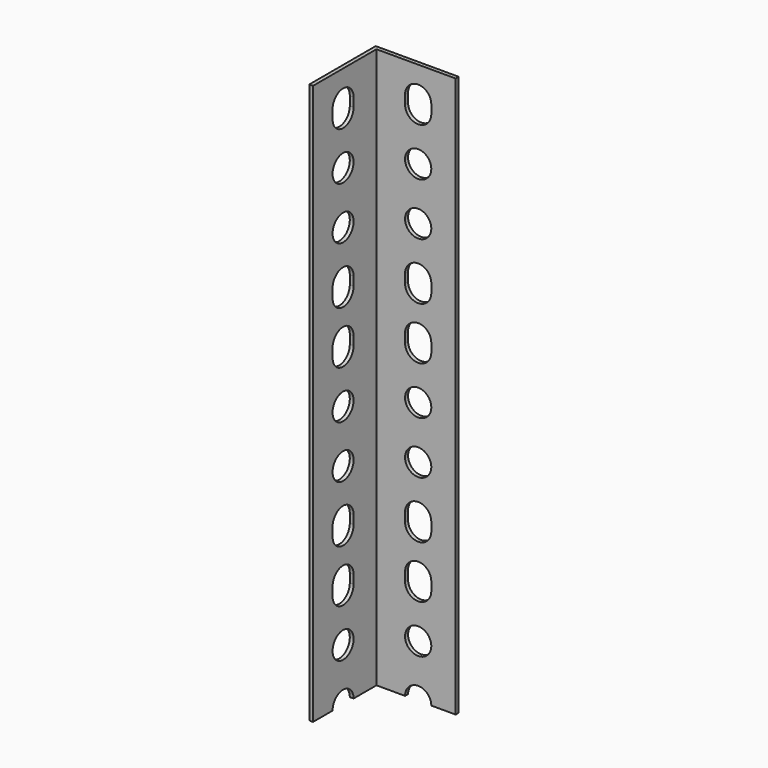
from build123d import *

# Parameters (mm, degrees)
F2_DEPTH = 203.2
F3_R     = 4.7625
F5_DEPTH = 1.3726
F4_R     = 4.7625
F6_DEPTH = 1.3726


# Not quite as in the source:
# - a variable given as a bare number and used for a length is read in inches; the dataset says mm whatever the document's units were


with BuildPart() as f2:
    # F1 (on Top) → F2 (new body)
    with BuildSketch(Plane.XY):
        Polygon((-1.3716, 1.3716), (-1.3716, -28.7528), (0, -28.7528), (0, 0), (28.7528, 0), (28.7528, 1.3716), align=None)
    extrude(amount=F2_DEPTH)

    # F3 (on face) → F5 (cut, through all)
    with BuildSketch(Plane.XZ):
        with Locations((15.1384, 19.05)):
            Circle(F3_R)
        with Locations((15.1384, 0)):
            Circle(F3_R)
        with BuildLine():
            Line((19.9009, 36.5125), (19.9009, 39.6875))
            ThreePointArc((19.9009, 39.6875), (15.1384, 44.45), (10.3759, 39.6875))
            Line((10.3759, 39.6875), (10.3759, 36.5125))
            ThreePointArc((10.3759, 36.5125), (15.1384, 31.75), (19.9009, 36.5125))
        make_face()
        with BuildLine():
            Line((19.9009, 55.5625), (19.9009, 58.7375))
            ThreePointArc((19.9009, 58.7375), (15.1384, 63.5), (10.3759, 58.7375))
            Line((10.3759, 58.7375), (10.3759, 55.5625))
            ThreePointArc((10.3759, 55.5625), (15.1384, 50.8), (19.9009, 55.5625))
        make_face()
        with BuildLine():
            Line((19.9009, 131.7625), (19.9009, 134.9375))
            ThreePointArc((19.9009, 134.9375), (15.1384, 139.7), (10.3759, 134.9375))
            Line((10.3759, 134.9375), (10.3759, 131.7625))
            ThreePointArc((10.3759, 131.7625), (15.1384, 127), (19.9009, 131.7625))
        make_face()
        with Locations((15.1384, 95.25)):
            Circle(F3_R)
        with Locations((15.1384, 76.2)):
            Circle(F3_R)
        with BuildLine():
            Line((19.9009, 112.7125), (19.9009, 115.8875))
            ThreePointArc((19.9009, 115.8875), (15.1384, 120.65), (10.3759, 115.8875))
            Line((10.3759, 115.8875), (10.3759, 112.7125))
            ThreePointArc((10.3759, 112.7125), (15.1384, 107.95), (19.9009, 112.7125))
        make_face()
        with BuildLine():
            Line((19.9009, 207.9625), (19.9009, 211.1375))
            ThreePointArc((19.9009, 211.1375), (15.1384, 215.9), (10.3759, 211.1375))
            Line((10.3759, 211.1375), (10.3759, 207.9625))
            ThreePointArc((10.3759, 207.9625), (15.1384, 203.2), (19.9009, 207.9625))
        make_face()
        with Locations((15.1384, 171.45)):
            Circle(F3_R)
        with Locations((15.1384, 152.4)):
            Circle(F3_R)
        with BuildLine():
            Line((19.9009, 188.9125), (19.9009, 192.0875))
            ThreePointArc((19.9009, 192.0875), (15.1384, 196.85), (10.3759, 192.0875))
            Line((10.3759, 192.0875), (10.3759, 188.9125))
            ThreePointArc((10.3759, 188.9125), (15.1384, 184.15), (19.9009, 188.9125))
        make_face()
        with BuildLine():
            Line((19.9009, 284.1625), (19.9009, 287.3375))
            ThreePointArc((19.9009, 287.3375), (15.1384, 292.1), (10.3759, 287.3375))
            Line((10.3759, 287.3375), (10.3759, 284.1625))
            ThreePointArc((10.3759, 284.1625), (15.1384, 279.4), (19.9009, 284.1625))
        make_face()
        with Locations((15.1384, 247.65)):
            Circle(F3_R)
        with Locations((15.1384, 228.6)):
            Circle(F3_R)
        with BuildLine():
            Line((19.9009, 265.1125), (19.9009, 268.2875))
            ThreePointArc((19.9009, 268.2875), (15.1384, 273.05), (10.3759, 268.2875))
            Line((10.3759, 268.2875), (10.3759, 265.1125))
            ThreePointArc((10.3759, 265.1125), (15.1384, 260.35), (19.9009, 265.1125))
        make_face()
        with BuildLine():
            Line((19.9009, 360.3625), (19.9009, 363.5375))
            ThreePointArc((19.9009, 363.5375), (15.1384, 368.3), (10.3759, 363.5375))
            Line((10.3759, 363.5375), (10.3759, 360.3625))
            ThreePointArc((10.3759, 360.3625), (15.1384, 355.6), (19.9009, 360.3625))
        make_face()
        with Locations((15.1384, 323.85)):
            Circle(F3_R)
        with Locations((15.1384, 304.8)):
            Circle(F3_R)
        with BuildLine():
            Line((19.9009, 341.3125), (19.9009, 344.4875))
            ThreePointArc((19.9009, 344.4875), (15.1384, 349.25), (10.3759, 344.4875))
            Line((10.3759, 344.4875), (10.3759, 341.3125))
            ThreePointArc((10.3759, 341.3125), (15.1384, 336.55), (19.9009, 341.3125))
        make_face()
        with BuildLine():
            Line((19.9009, 436.5625), (19.9009, 439.7375))
            ThreePointArc((19.9009, 439.7375), (15.1384, 444.5), (10.3759, 439.7375))
            Line((10.3759, 439.7375), (10.3759, 436.5625))
            ThreePointArc((10.3759, 436.5625), (15.1384, 431.8), (19.9009, 436.5625))
        make_face()
        with Locations((15.1384, 400.05)):
            Circle(F3_R)
        with Locations((15.1384, 381)):
            Circle(F3_R)
        with BuildLine():
            Line((19.9009, 417.5125), (19.9009, 420.6875))
            ThreePointArc((19.9009, 420.6875), (15.1384, 425.45), (10.3759, 420.6875))
            Line((10.3759, 420.6875), (10.3759, 417.5125))
            ThreePointArc((10.3759, 417.5125), (15.1384, 412.75), (19.9009, 417.5125))
        make_face()
        with BuildLine():
            Line((19.9009, 512.7625), (19.9009, 515.9375))
            ThreePointArc((19.9009, 515.9375), (15.1384, 520.7), (10.3759, 515.9375))
            Line((10.3759, 515.9375), (10.3759, 512.7625))
            ThreePointArc((10.3759, 512.7625), (15.1384, 508), (19.9009, 512.7625))
        make_face()
        with Locations((15.1384, 476.25)):
            Circle(F3_R)
        with Locations((15.1384, 457.2)):
            Circle(F3_R)
        with BuildLine():
            Line((19.9009, 493.7125), (19.9009, 496.8875))
            ThreePointArc((19.9009, 496.8875), (15.1384, 501.65), (10.3759, 496.8875))
            Line((10.3759, 496.8875), (10.3759, 493.7125))
            ThreePointArc((10.3759, 493.7125), (15.1384, 488.95), (19.9009, 493.7125))
        make_face()
        with BuildLine():
            Line((19.9009, 588.9625), (19.9009, 592.1375))
            ThreePointArc((19.9009, 592.1375), (15.1384, 596.9), (10.3759, 592.1375))
            Line((10.3759, 592.1375), (10.3759, 588.9625))
            ThreePointArc((10.3759, 588.9625), (15.1384, 584.2), (19.9009, 588.9625))
        make_face()
        with Locations((15.1384, 552.45)):
            Circle(F3_R)
        with Locations((15.1384, 533.4)):
            Circle(F3_R)
        with BuildLine():
            Line((19.9009, 569.9125), (19.9009, 573.0875))
            ThreePointArc((19.9009, 573.0875), (15.1384, 577.85), (10.3759, 573.0875))
            Line((10.3759, 573.0875), (10.3759, 569.9125))
            ThreePointArc((10.3759, 569.9125), (15.1384, 565.15), (19.9009, 569.9125))
        make_face()
        with BuildLine():
            Line((19.9009, 665.1625), (19.9009, 668.3375))
            ThreePointArc((19.9009, 668.3375), (15.1384, 673.1), (10.3759, 668.3375))
            Line((10.3759, 668.3375), (10.3759, 665.1625))
            ThreePointArc((10.3759, 665.1625), (15.1384, 660.4), (19.9009, 665.1625))
        make_face()
        with Locations((15.1384, 628.65)):
            Circle(F3_R)
        with Locations((15.1384, 609.6)):
            Circle(F3_R)
        with BuildLine():
            Line((19.9009, 646.1125), (19.9009, 649.2875))
            ThreePointArc((19.9009, 649.2875), (15.1384, 654.05), (10.3759, 649.2875))
            Line((10.3759, 649.2875), (10.3759, 646.1125))
            ThreePointArc((10.3759, 646.1125), (15.1384, 641.35), (19.9009, 646.1125))
        make_face()
        with BuildLine():
            Line((19.9009, 741.3625), (19.9009, 744.5375))
            ThreePointArc((19.9009, 744.5375), (15.1384, 749.3), (10.3759, 744.5375))
            Line((10.3759, 744.5375), (10.3759, 741.3625))
            ThreePointArc((10.3759, 741.3625), (15.1384, 736.6), (19.9009, 741.3625))
        make_face()
        with Locations((15.1384, 704.85)):
            Circle(F3_R)
        with Locations((15.1384, 685.8)):
            Circle(F3_R)
        with BuildLine():
            Line((19.9009, 722.3125), (19.9009, 725.4875))
            ThreePointArc((19.9009, 725.4875), (15.1384, 730.25), (10.3759, 725.4875))
            Line((10.3759, 725.4875), (10.3759, 722.3125))
            ThreePointArc((10.3759, 722.3125), (15.1384, 717.55), (19.9009, 722.3125))
        make_face()
        with BuildLine():
            Line((19.9009, 817.5625), (19.9009, 820.7375))
            ThreePointArc((19.9009, 820.7375), (15.1384, 825.5), (10.3759, 820.7375))
            Line((10.3759, 820.7375), (10.3759, 817.5625))
            ThreePointArc((10.3759, 817.5625), (15.1384, 812.8), (19.9009, 817.5625))
        make_face()
        with Locations((15.1384, 781.05)):
            Circle(F3_R)
        with Locations((15.1384, 762)):
            Circle(F3_R)
        with BuildLine():
            Line((19.9009, 798.5125), (19.9009, 801.6875))
            ThreePointArc((19.9009, 801.6875), (15.1384, 806.45), (10.3759, 801.6875))
            Line((10.3759, 801.6875), (10.3759, 798.5125))
            ThreePointArc((10.3759, 798.5125), (15.1384, 793.75), (19.9009, 798.5125))
        make_face()
        with BuildLine():
            Line((19.9009, 893.7625), (19.9009, 896.9375))
            ThreePointArc((19.9009, 896.9375), (15.1384, 901.7), (10.3759, 896.9375))
            Line((10.3759, 896.9375), (10.3759, 893.7625))
            ThreePointArc((10.3759, 893.7625), (15.1384, 889), (19.9009, 893.7625))
        make_face()
        with Locations((15.1384, 857.25)):
            Circle(F3_R)
        with Locations((15.1384, 838.2)):
            Circle(F3_R)
        with BuildLine():
            Line((19.9009, 874.7125), (19.9009, 877.8875))
            ThreePointArc((19.9009, 877.8875), (15.1384, 882.65), (10.3759, 877.8875))
            Line((10.3759, 877.8875), (10.3759, 874.7125))
            ThreePointArc((10.3759, 874.7125), (15.1384, 869.95), (19.9009, 874.7125))
        make_face()
        with BuildLine():
            Line((19.9009, 969.9625), (19.9009, 973.1375))
            ThreePointArc((19.9009, 973.1375), (15.1384, 977.9), (10.3759, 973.1375))
            Line((10.3759, 973.1375), (10.3759, 969.9625))
            ThreePointArc((10.3759, 969.9625), (15.1384, 965.2), (19.9009, 969.9625))
        make_face()
        with Locations((15.1384, 933.45)):
            Circle(F3_R)
        with Locations((15.1384, 914.4)):
            Circle(F3_R)
        with BuildLine():
            Line((19.9009, 950.9125), (19.9009, 954.0875))
            ThreePointArc((19.9009, 954.0875), (15.1384, 958.85), (10.3759, 954.0875))
            Line((10.3759, 954.0875), (10.3759, 950.9125))
            ThreePointArc((10.3759, 950.9125), (15.1384, 946.15), (19.9009, 950.9125))
        make_face()
        with BuildLine():
            Line((19.9009, 1046.1625), (19.9009, 1049.3375))
            ThreePointArc((19.9009, 1049.3375), (15.1384, 1054.1), (10.3759, 1049.3375))
            Line((10.3759, 1049.3375), (10.3759, 1046.1625))
            ThreePointArc((10.3759, 1046.1625), (15.1384, 1041.4), (19.9009, 1046.1625))
        make_face()
        with Locations((15.1384, 1009.65)):
            Circle(F3_R)
        with Locations((15.1384, 990.6)):
            Circle(F3_R)
        with BuildLine():
            Line((19.9009, 1027.1125), (19.9009, 1030.2875))
            ThreePointArc((19.9009, 1030.2875), (15.1384, 1035.05), (10.3759, 1030.2875))
            Line((10.3759, 1030.2875), (10.3759, 1027.1125))
            ThreePointArc((10.3759, 1027.1125), (15.1384, 1022.35), (19.9009, 1027.1125))
        make_face()
        with BuildLine():
            Line((19.9009, 1122.3625), (19.9009, 1125.5375))
            ThreePointArc((19.9009, 1125.5375), (15.1384, 1130.3), (10.3759, 1125.5375))
            Line((10.3759, 1125.5375), (10.3759, 1122.3625))
            ThreePointArc((10.3759, 1122.3625), (15.1384, 1117.6), (19.9009, 1122.3625))
        make_face()
        with Locations((15.1384, 1085.85)):
            Circle(F3_R)
        with Locations((15.1384, 1066.8)):
            Circle(F3_R)
        with BuildLine():
            Line((19.9009, 1103.3125), (19.9009, 1106.4875))
            ThreePointArc((19.9009, 1106.4875), (15.1384, 1111.25), (10.3759, 1106.4875))
            Line((10.3759, 1106.4875), (10.3759, 1103.3125))
            ThreePointArc((10.3759, 1103.3125), (15.1384, 1098.55), (19.9009, 1103.3125))
        make_face()
        with BuildLine():
            Line((19.9009, 1198.5625), (19.9009, 1201.7375))
            ThreePointArc((19.9009, 1201.7375), (15.1384, 1206.5), (10.3759, 1201.7375))
            Line((10.3759, 1201.7375), (10.3759, 1198.5625))
            ThreePointArc((10.3759, 1198.5625), (15.1384, 1193.8), (19.9009, 1198.5625))
        make_face()
        with Locations((15.1384, 1162.05)):
            Circle(F3_R)
        with Locations((15.1384, 1143)):
            Circle(F3_R)
        with BuildLine():
            Line((19.9009, 1179.5125), (19.9009, 1182.6875))
            ThreePointArc((19.9009, 1182.6875), (15.1384, 1187.45), (10.3759, 1182.6875))
            Line((10.3759, 1182.6875), (10.3759, 1179.5125))
            ThreePointArc((10.3759, 1179.5125), (15.1384, 1174.75), (19.9009, 1179.5125))
        make_face()
        with BuildLine():
            Line((19.9009, 1274.7625), (19.9009, 1277.9375))
            ThreePointArc((19.9009, 1277.9375), (15.1384, 1282.7), (10.3759, 1277.9375))
            Line((10.3759, 1277.9375), (10.3759, 1274.7625))
            ThreePointArc((10.3759, 1274.7625), (15.1384, 1270), (19.9009, 1274.7625))
        make_face()
        with Locations((15.1384, 1238.25)):
            Circle(F3_R)
        with Locations((15.1384, 1219.2)):
            Circle(F3_R)
        with BuildLine():
            Line((19.9009, 1255.7125), (19.9009, 1258.8875))
            ThreePointArc((19.9009, 1258.8875), (15.1384, 1263.65), (10.3759, 1258.8875))
            Line((10.3759, 1258.8875), (10.3759, 1255.7125))
            ThreePointArc((10.3759, 1255.7125), (15.1384, 1250.95), (19.9009, 1255.7125))
        make_face()
        with BuildLine():
            Line((19.9009, 1350.9625), (19.9009, 1354.1375))
            ThreePointArc((19.9009, 1354.1375), (15.1384, 1358.9), (10.3759, 1354.1375))
            Line((10.3759, 1354.1375), (10.3759, 1350.9625))
            ThreePointArc((10.3759, 1350.9625), (15.1384, 1346.2), (19.9009, 1350.9625))
        make_face()
        with Locations((15.1384, 1314.45)):
            Circle(F3_R)
        with Locations((15.1384, 1295.4)):
            Circle(F3_R)
        with BuildLine():
            Line((19.9009, 1331.9125), (19.9009, 1335.0875))
            ThreePointArc((19.9009, 1335.0875), (15.1384, 1339.85), (10.3759, 1335.0875))
            Line((10.3759, 1335.0875), (10.3759, 1331.9125))
            ThreePointArc((10.3759, 1331.9125), (15.1384, 1327.15), (19.9009, 1331.9125))
        make_face()
        with BuildLine():
            Line((19.9009, 1427.1625), (19.9009, 1430.3375))
            ThreePointArc((19.9009, 1430.3375), (15.1384, 1435.1), (10.3759, 1430.3375))
            Line((10.3759, 1430.3375), (10.3759, 1427.1625))
            ThreePointArc((10.3759, 1427.1625), (15.1384, 1422.4), (19.9009, 1427.1625))
        make_face()
        with Locations((15.1384, 1390.65)):
            Circle(F3_R)
        with Locations((15.1384, 1371.6)):
            Circle(F3_R)
        with BuildLine():
            Line((19.9009, 1408.1125), (19.9009, 1411.2875))
            ThreePointArc((19.9009, 1411.2875), (15.1384, 1416.05), (10.3759, 1411.2875))
            Line((10.3759, 1411.2875), (10.3759, 1408.1125))
            ThreePointArc((10.3759, 1408.1125), (15.1384, 1403.35), (19.9009, 1408.1125))
        make_face()
        with BuildLine():
            Line((19.9009, 1503.3625), (19.9009, 1506.5375))
            ThreePointArc((19.9009, 1506.5375), (15.1384, 1511.3), (10.3759, 1506.5375))
            Line((10.3759, 1506.5375), (10.3759, 1503.3625))
            ThreePointArc((10.3759, 1503.3625), (15.1384, 1498.6), (19.9009, 1503.3625))
        make_face()
        with Locations((15.1384, 1466.85)):
            Circle(F3_R)
        with Locations((15.1384, 1447.8)):
            Circle(F3_R)
        with BuildLine():
            Line((19.9009, 1484.3125), (19.9009, 1487.4875))
            ThreePointArc((19.9009, 1487.4875), (15.1384, 1492.25), (10.3759, 1487.4875))
            Line((10.3759, 1487.4875), (10.3759, 1484.3125))
            ThreePointArc((10.3759, 1484.3125), (15.1384, 1479.55), (19.9009, 1484.3125))
        make_face()
        with BuildLine():
            Line((19.9009, 1579.5625), (19.9009, 1582.7375))
            ThreePointArc((19.9009, 1582.7375), (15.1384, 1587.5), (10.3759, 1582.7375))
            Line((10.3759, 1582.7375), (10.3759, 1579.5625))
            ThreePointArc((10.3759, 1579.5625), (15.1384, 1574.8), (19.9009, 1579.5625))
        make_face()
        with Locations((15.1384, 1543.05)):
            Circle(F3_R)
        with Locations((15.1384, 1524)):
            Circle(F3_R)
        with BuildLine():
            Line((19.9009, 1560.5125), (19.9009, 1563.6875))
            ThreePointArc((19.9009, 1563.6875), (15.1384, 1568.45), (10.3759, 1563.6875))
            Line((10.3759, 1563.6875), (10.3759, 1560.5125))
            ThreePointArc((10.3759, 1560.5125), (15.1384, 1555.75), (19.9009, 1560.5125))
        make_face()
        with BuildLine():
            Line((19.9009, 1655.7625), (19.9009, 1658.9375))
            ThreePointArc((19.9009, 1658.9375), (15.1384, 1663.7), (10.3759, 1658.9375))
            Line((10.3759, 1658.9375), (10.3759, 1655.7625))
            ThreePointArc((10.3759, 1655.7625), (15.1384, 1651), (19.9009, 1655.7625))
        make_face()
        with Locations((15.1384, 1619.25)):
            Circle(F3_R)
        with Locations((15.1384, 1600.2)):
            Circle(F3_R)
        with BuildLine():
            Line((19.9009, 1636.7125), (19.9009, 1639.8875))
            ThreePointArc((19.9009, 1639.8875), (15.1384, 1644.65), (10.3759, 1639.8875))
            Line((10.3759, 1639.8875), (10.3759, 1636.7125))
            ThreePointArc((10.3759, 1636.7125), (15.1384, 1631.95), (19.9009, 1636.7125))
        make_face()
        with BuildLine():
            Line((19.9009, 1731.9625), (19.9009, 1735.1375))
            ThreePointArc((19.9009, 1735.1375), (15.1384, 1739.9), (10.3759, 1735.1375))
            Line((10.3759, 1735.1375), (10.3759, 1731.9625))
            ThreePointArc((10.3759, 1731.9625), (15.1384, 1727.2), (19.9009, 1731.9625))
        make_face()
        with Locations((15.1384, 1695.45)):
            Circle(F3_R)
        with Locations((15.1384, 1676.4)):
            Circle(F3_R)
        with BuildLine():
            Line((19.9009, 1712.9125), (19.9009, 1716.0875))
            ThreePointArc((19.9009, 1716.0875), (15.1384, 1720.85), (10.3759, 1716.0875))
            Line((10.3759, 1716.0875), (10.3759, 1712.9125))
            ThreePointArc((10.3759, 1712.9125), (15.1384, 1708.15), (19.9009, 1712.9125))
        make_face()
        with BuildLine():
            Line((19.9009, 1808.1625), (19.9009, 1811.3375))
            ThreePointArc((19.9009, 1811.3375), (15.1384, 1816.1), (10.3759, 1811.3375))
            Line((10.3759, 1811.3375), (10.3759, 1808.1625))
            ThreePointArc((10.3759, 1808.1625), (15.1384, 1803.4), (19.9009, 1808.1625))
        make_face()
        with Locations((15.1384, 1771.65)):
            Circle(F3_R)
        with Locations((15.1384, 1752.6)):
            Circle(F3_R)
        with BuildLine():
            Line((19.9009, 1789.1125), (19.9009, 1792.2875))
            ThreePointArc((19.9009, 1792.2875), (15.1384, 1797.05), (10.3759, 1792.2875))
            Line((10.3759, 1792.2875), (10.3759, 1789.1125))
            ThreePointArc((10.3759, 1789.1125), (15.1384, 1784.35), (19.9009, 1789.1125))
        make_face()
    extrude(amount=-F5_DEPTH, mode=Mode.SUBTRACT)

    # F4 (on face) → F6 (cut, through all)
    with BuildSketch(Plane.YZ):
        with Locations((-15.1384, 19.05)):
            Circle(F4_R)
        with Locations((-15.1384, 0)):
            Circle(F4_R)
        with BuildLine():
            Line((-10.3759, 36.5125), (-10.3759, 39.6875))
            ThreePointArc((-10.3759, 39.6875), (-15.1384, 44.45), (-19.9009, 39.6875))
            Line((-19.9009, 39.6875), (-19.9009, 36.5125))
            ThreePointArc((-19.9009, 36.5125), (-15.1384, 31.75), (-10.3759, 36.5125))
        make_face()
        with BuildLine():
            Line((-10.3759, 55.5625), (-10.3759, 58.7375))
            ThreePointArc((-10.3759, 58.7375), (-15.1384, 63.5), (-19.9009, 58.7375))
            Line((-19.9009, 58.7375), (-19.9009, 55.5625))
            ThreePointArc((-19.9009, 55.5625), (-15.1384, 50.8), (-10.3759, 55.5625))
        make_face()
        with BuildLine():
            Line((-10.3759, 131.7625), (-10.3759, 134.9375))
            ThreePointArc((-10.3759, 134.9375), (-15.1384, 139.7), (-19.9009, 134.9375))
            Line((-19.9009, 134.9375), (-19.9009, 131.7625))
            ThreePointArc((-19.9009, 131.7625), (-15.1384, 127), (-10.3759, 131.7625))
        make_face()
        with Locations((-15.1384, 95.25)):
            Circle(F4_R)
        with Locations((-15.1384, 76.2)):
            Circle(F4_R)
        with BuildLine():
            Line((-10.3759, 112.7125), (-10.3759, 115.8875))
            ThreePointArc((-10.3759, 115.8875), (-15.1384, 120.65), (-19.9009, 115.8875))
            Line((-19.9009, 115.8875), (-19.9009, 112.7125))
            ThreePointArc((-19.9009, 112.7125), (-15.1384, 107.95), (-10.3759, 112.7125))
        make_face()
        with BuildLine():
            Line((-10.3759, 207.9625), (-10.3759, 211.1375))
            ThreePointArc((-10.3759, 211.1375), (-15.1384, 215.9), (-19.9009, 211.1375))
            Line((-19.9009, 211.1375), (-19.9009, 207.9625))
            ThreePointArc((-19.9009, 207.9625), (-15.1384, 203.2), (-10.3759, 207.9625))
        make_face()
        with Locations((-15.1384, 171.45)):
            Circle(F4_R)
        with Locations((-15.1384, 152.4)):
            Circle(F4_R)
        with BuildLine():
            Line((-10.3759, 188.9125), (-10.3759, 192.0875))
            ThreePointArc((-10.3759, 192.0875), (-15.1384, 196.85), (-19.9009, 192.0875))
            Line((-19.9009, 192.0875), (-19.9009, 188.9125))
            ThreePointArc((-19.9009, 188.9125), (-15.1384, 184.15), (-10.3759, 188.9125))
        make_face()
        with BuildLine():
            Line((-10.3759, 284.1625), (-10.3759, 287.3375))
            ThreePointArc((-10.3759, 287.3375), (-15.1384, 292.1), (-19.9009, 287.3375))
            Line((-19.9009, 287.3375), (-19.9009, 284.1625))
            ThreePointArc((-19.9009, 284.1625), (-15.1384, 279.4), (-10.3759, 284.1625))
        make_face()
        with Locations((-15.1384, 247.65)):
            Circle(F4_R)
        with Locations((-15.1384, 228.6)):
            Circle(F4_R)
        with BuildLine():
            Line((-10.3759, 265.1125), (-10.3759, 268.2875))
            ThreePointArc((-10.3759, 268.2875), (-15.1384, 273.05), (-19.9009, 268.2875))
            Line((-19.9009, 268.2875), (-19.9009, 265.1125))
            ThreePointArc((-19.9009, 265.1125), (-15.1384, 260.35), (-10.3759, 265.1125))
        make_face()
        with BuildLine():
            Line((-10.3759, 360.3625), (-10.3759, 363.5375))
            ThreePointArc((-10.3759, 363.5375), (-15.1384, 368.3), (-19.9009, 363.5375))
            Line((-19.9009, 363.5375), (-19.9009, 360.3625))
            ThreePointArc((-19.9009, 360.3625), (-15.1384, 355.6), (-10.3759, 360.3625))
        make_face()
        with Locations((-15.1384, 323.85)):
            Circle(F4_R)
        with Locations((-15.1384, 304.8)):
            Circle(F4_R)
        with BuildLine():
            Line((-10.3759, 341.3125), (-10.3759, 344.4875))
            ThreePointArc((-10.3759, 344.4875), (-15.1384, 349.25), (-19.9009, 344.4875))
            Line((-19.9009, 344.4875), (-19.9009, 341.3125))
            ThreePointArc((-19.9009, 341.3125), (-15.1384, 336.55), (-10.3759, 341.3125))
        make_face()
        with BuildLine():
            Line((-10.3759, 436.5625), (-10.3759, 439.7375))
            ThreePointArc((-10.3759, 439.7375), (-15.1384, 444.5), (-19.9009, 439.7375))
            Line((-19.9009, 439.7375), (-19.9009, 436.5625))
            ThreePointArc((-19.9009, 436.5625), (-15.1384, 431.8), (-10.3759, 436.5625))
        make_face()
        with Locations((-15.1384, 400.05)):
            Circle(F4_R)
        with Locations((-15.1384, 381)):
            Circle(F4_R)
        with BuildLine():
            Line((-10.3759, 417.5125), (-10.3759, 420.6875))
            ThreePointArc((-10.3759, 420.6875), (-15.1384, 425.45), (-19.9009, 420.6875))
            Line((-19.9009, 420.6875), (-19.9009, 417.5125))
            ThreePointArc((-19.9009, 417.5125), (-15.1384, 412.75), (-10.3759, 417.5125))
        make_face()
        with BuildLine():
            Line((-10.3759, 512.7625), (-10.3759, 515.9375))
            ThreePointArc((-10.3759, 515.9375), (-15.1384, 520.7), (-19.9009, 515.9375))
            Line((-19.9009, 515.9375), (-19.9009, 512.7625))
            ThreePointArc((-19.9009, 512.7625), (-15.1384, 508), (-10.3759, 512.7625))
        make_face()
        with Locations((-15.1384, 476.25)):
            Circle(F4_R)
        with Locations((-15.1384, 457.2)):
            Circle(F4_R)
        with BuildLine():
            Line((-10.3759, 493.7125), (-10.3759, 496.8875))
            ThreePointArc((-10.3759, 496.8875), (-15.1384, 501.65), (-19.9009, 496.8875))
            Line((-19.9009, 496.8875), (-19.9009, 493.7125))
            ThreePointArc((-19.9009, 493.7125), (-15.1384, 488.95), (-10.3759, 493.7125))
        make_face()
        with BuildLine():
            Line((-10.3759, 588.9625), (-10.3759, 592.1375))
            ThreePointArc((-10.3759, 592.1375), (-15.1384, 596.9), (-19.9009, 592.1375))
            Line((-19.9009, 592.1375), (-19.9009, 588.9625))
            ThreePointArc((-19.9009, 588.9625), (-15.1384, 584.2), (-10.3759, 588.9625))
        make_face()
        with Locations((-15.1384, 552.45)):
            Circle(F4_R)
        with Locations((-15.1384, 533.4)):
            Circle(F4_R)
        with BuildLine():
            Line((-10.3759, 569.9125), (-10.3759, 573.0875))
            ThreePointArc((-10.3759, 573.0875), (-15.1384, 577.85), (-19.9009, 573.0875))
            Line((-19.9009, 573.0875), (-19.9009, 569.9125))
            ThreePointArc((-19.9009, 569.9125), (-15.1384, 565.15), (-10.3759, 569.9125))
        make_face()
        with BuildLine():
            Line((-10.3759, 665.1625), (-10.3759, 668.3375))
            ThreePointArc((-10.3759, 668.3375), (-15.1384, 673.1), (-19.9009, 668.3375))
            Line((-19.9009, 668.3375), (-19.9009, 665.1625))
            ThreePointArc((-19.9009, 665.1625), (-15.1384, 660.4), (-10.3759, 665.1625))
        make_face()
        with Locations((-15.1384, 628.65)):
            Circle(F4_R)
        with Locations((-15.1384, 609.6)):
            Circle(F4_R)
        with BuildLine():
            Line((-10.3759, 646.1125), (-10.3759, 649.2875))
            ThreePointArc((-10.3759, 649.2875), (-15.1384, 654.05), (-19.9009, 649.2875))
            Line((-19.9009, 649.2875), (-19.9009, 646.1125))
            ThreePointArc((-19.9009, 646.1125), (-15.1384, 641.35), (-10.3759, 646.1125))
        make_face()
        with BuildLine():
            Line((-10.3759, 741.3625), (-10.3759, 744.5375))
            ThreePointArc((-10.3759, 744.5375), (-15.1384, 749.3), (-19.9009, 744.5375))
            Line((-19.9009, 744.5375), (-19.9009, 741.3625))
            ThreePointArc((-19.9009, 741.3625), (-15.1384, 736.6), (-10.3759, 741.3625))
        make_face()
        with Locations((-15.1384, 704.85)):
            Circle(F4_R)
        with Locations((-15.1384, 685.8)):
            Circle(F4_R)
        with BuildLine():
            Line((-10.3759, 722.3125), (-10.3759, 725.4875))
            ThreePointArc((-10.3759, 725.4875), (-15.1384, 730.25), (-19.9009, 725.4875))
            Line((-19.9009, 725.4875), (-19.9009, 722.3125))
            ThreePointArc((-19.9009, 722.3125), (-15.1384, 717.55), (-10.3759, 722.3125))
        make_face()
        with BuildLine():
            Line((-10.3759, 817.5625), (-10.3759, 820.7375))
            ThreePointArc((-10.3759, 820.7375), (-15.1384, 825.5), (-19.9009, 820.7375))
            Line((-19.9009, 820.7375), (-19.9009, 817.5625))
            ThreePointArc((-19.9009, 817.5625), (-15.1384, 812.8), (-10.3759, 817.5625))
        make_face()
        with Locations((-15.1384, 781.05)):
            Circle(F4_R)
        with Locations((-15.1384, 762)):
            Circle(F4_R)
        with BuildLine():
            Line((-10.3759, 798.5125), (-10.3759, 801.6875))
            ThreePointArc((-10.3759, 801.6875), (-15.1384, 806.45), (-19.9009, 801.6875))
            Line((-19.9009, 801.6875), (-19.9009, 798.5125))
            ThreePointArc((-19.9009, 798.5125), (-15.1384, 793.75), (-10.3759, 798.5125))
        make_face()
        with BuildLine():
            Line((-10.3759, 893.7625), (-10.3759, 896.9375))
            ThreePointArc((-10.3759, 896.9375), (-15.1384, 901.7), (-19.9009, 896.9375))
            Line((-19.9009, 896.9375), (-19.9009, 893.7625))
            ThreePointArc((-19.9009, 893.7625), (-15.1384, 889), (-10.3759, 893.7625))
        make_face()
        with Locations((-15.1384, 857.25)):
            Circle(F4_R)
        with Locations((-15.1384, 838.2)):
            Circle(F4_R)
        with BuildLine():
            Line((-10.3759, 874.7125), (-10.3759, 877.8875))
            ThreePointArc((-10.3759, 877.8875), (-15.1384, 882.65), (-19.9009, 877.8875))
            Line((-19.9009, 877.8875), (-19.9009, 874.7125))
            ThreePointArc((-19.9009, 874.7125), (-15.1384, 869.95), (-10.3759, 874.7125))
        make_face()
        with BuildLine():
            Line((-10.3759, 969.9625), (-10.3759, 973.1375))
            ThreePointArc((-10.3759, 973.1375), (-15.1384, 977.9), (-19.9009, 973.1375))
            Line((-19.9009, 973.1375), (-19.9009, 969.9625))
            ThreePointArc((-19.9009, 969.9625), (-15.1384, 965.2), (-10.3759, 969.9625))
        make_face()
        with Locations((-15.1384, 933.45)):
            Circle(F4_R)
        with Locations((-15.1384, 914.4)):
            Circle(F4_R)
        with BuildLine():
            Line((-10.3759, 950.9125), (-10.3759, 954.0875))
            ThreePointArc((-10.3759, 954.0875), (-15.1384, 958.85), (-19.9009, 954.0875))
            Line((-19.9009, 954.0875), (-19.9009, 950.9125))
            ThreePointArc((-19.9009, 950.9125), (-15.1384, 946.15), (-10.3759, 950.9125))
        make_face()
        with BuildLine():
            Line((-10.3759, 1046.1625), (-10.3759, 1049.3375))
            ThreePointArc((-10.3759, 1049.3375), (-15.1384, 1054.1), (-19.9009, 1049.3375))
            Line((-19.9009, 1049.3375), (-19.9009, 1046.1625))
            ThreePointArc((-19.9009, 1046.1625), (-15.1384, 1041.4), (-10.3759, 1046.1625))
        make_face()
        with Locations((-15.1384, 1009.65)):
            Circle(F4_R)
        with Locations((-15.1384, 990.6)):
            Circle(F4_R)
        with BuildLine():
            Line((-10.3759, 1027.1125), (-10.3759, 1030.2875))
            ThreePointArc((-10.3759, 1030.2875), (-15.1384, 1035.05), (-19.9009, 1030.2875))
            Line((-19.9009, 1030.2875), (-19.9009, 1027.1125))
            ThreePointArc((-19.9009, 1027.1125), (-15.1384, 1022.35), (-10.3759, 1027.1125))
        make_face()
        with BuildLine():
            Line((-10.3759, 1122.3625), (-10.3759, 1125.5375))
            ThreePointArc((-10.3759, 1125.5375), (-15.1384, 1130.3), (-19.9009, 1125.5375))
            Line((-19.9009, 1125.5375), (-19.9009, 1122.3625))
            ThreePointArc((-19.9009, 1122.3625), (-15.1384, 1117.6), (-10.3759, 1122.3625))
        make_face()
        with Locations((-15.1384, 1085.85)):
            Circle(F4_R)
        with Locations((-15.1384, 1066.8)):
            Circle(F4_R)
        with BuildLine():
            Line((-10.3759, 1103.3125), (-10.3759, 1106.4875))
            ThreePointArc((-10.3759, 1106.4875), (-15.1384, 1111.25), (-19.9009, 1106.4875))
            Line((-19.9009, 1106.4875), (-19.9009, 1103.3125))
            ThreePointArc((-19.9009, 1103.3125), (-15.1384, 1098.55), (-10.3759, 1103.3125))
        make_face()
        with BuildLine():
            Line((-10.3759, 1198.5625), (-10.3759, 1201.7375))
            ThreePointArc((-10.3759, 1201.7375), (-15.1384, 1206.5), (-19.9009, 1201.7375))
            Line((-19.9009, 1201.7375), (-19.9009, 1198.5625))
            ThreePointArc((-19.9009, 1198.5625), (-15.1384, 1193.8), (-10.3759, 1198.5625))
        make_face()
        with Locations((-15.1384, 1162.05)):
            Circle(F4_R)
        with Locations((-15.1384, 1143)):
            Circle(F4_R)
        with BuildLine():
            Line((-10.3759, 1179.5125), (-10.3759, 1182.6875))
            ThreePointArc((-10.3759, 1182.6875), (-15.1384, 1187.45), (-19.9009, 1182.6875))
            Line((-19.9009, 1182.6875), (-19.9009, 1179.5125))
            ThreePointArc((-19.9009, 1179.5125), (-15.1384, 1174.75), (-10.3759, 1179.5125))
        make_face()
        with BuildLine():
            Line((-10.3759, 1274.7625), (-10.3759, 1277.9375))
            ThreePointArc((-10.3759, 1277.9375), (-15.1384, 1282.7), (-19.9009, 1277.9375))
            Line((-19.9009, 1277.9375), (-19.9009, 1274.7625))
            ThreePointArc((-19.9009, 1274.7625), (-15.1384, 1270), (-10.3759, 1274.7625))
        make_face()
        with Locations((-15.1384, 1238.25)):
            Circle(F4_R)
        with Locations((-15.1384, 1219.2)):
            Circle(F4_R)
        with BuildLine():
            Line((-10.3759, 1255.7125), (-10.3759, 1258.8875))
            ThreePointArc((-10.3759, 1258.8875), (-15.1384, 1263.65), (-19.9009, 1258.8875))
            Line((-19.9009, 1258.8875), (-19.9009, 1255.7125))
            ThreePointArc((-19.9009, 1255.7125), (-15.1384, 1250.95), (-10.3759, 1255.7125))
        make_face()
        with BuildLine():
            Line((-10.3759, 1350.9625), (-10.3759, 1354.1375))
            ThreePointArc((-10.3759, 1354.1375), (-15.1384, 1358.9), (-19.9009, 1354.1375))
            Line((-19.9009, 1354.1375), (-19.9009, 1350.9625))
            ThreePointArc((-19.9009, 1350.9625), (-15.1384, 1346.2), (-10.3759, 1350.9625))
        make_face()
        with Locations((-15.1384, 1314.45)):
            Circle(F4_R)
        with Locations((-15.1384, 1295.4)):
            Circle(F4_R)
        with BuildLine():
            Line((-10.3759, 1331.9125), (-10.3759, 1335.0875))
            ThreePointArc((-10.3759, 1335.0875), (-15.1384, 1339.85), (-19.9009, 1335.0875))
            Line((-19.9009, 1335.0875), (-19.9009, 1331.9125))
            ThreePointArc((-19.9009, 1331.9125), (-15.1384, 1327.15), (-10.3759, 1331.9125))
        make_face()
        with BuildLine():
            Line((-10.3759, 1427.1625), (-10.3759, 1430.3375))
            ThreePointArc((-10.3759, 1430.3375), (-15.1384, 1435.1), (-19.9009, 1430.3375))
            Line((-19.9009, 1430.3375), (-19.9009, 1427.1625))
            ThreePointArc((-19.9009, 1427.1625), (-15.1384, 1422.4), (-10.3759, 1427.1625))
        make_face()
        with Locations((-15.1384, 1390.65)):
            Circle(F4_R)
        with Locations((-15.1384, 1371.6)):
            Circle(F4_R)
        with BuildLine():
            Line((-10.3759, 1408.1125), (-10.3759, 1411.2875))
            ThreePointArc((-10.3759, 1411.2875), (-15.1384, 1416.05), (-19.9009, 1411.2875))
            Line((-19.9009, 1411.2875), (-19.9009, 1408.1125))
            ThreePointArc((-19.9009, 1408.1125), (-15.1384, 1403.35), (-10.3759, 1408.1125))
        make_face()
        with BuildLine():
            Line((-10.3759, 1503.3625), (-10.3759, 1506.5375))
            ThreePointArc((-10.3759, 1506.5375), (-15.1384, 1511.3), (-19.9009, 1506.5375))
            Line((-19.9009, 1506.5375), (-19.9009, 1503.3625))
            ThreePointArc((-19.9009, 1503.3625), (-15.1384, 1498.6), (-10.3759, 1503.3625))
        make_face()
        with Locations((-15.1384, 1466.85)):
            Circle(F4_R)
        with Locations((-15.1384, 1447.8)):
            Circle(F4_R)
        with BuildLine():
            Line((-10.3759, 1484.3125), (-10.3759, 1487.4875))
            ThreePointArc((-10.3759, 1487.4875), (-15.1384, 1492.25), (-19.9009, 1487.4875))
            Line((-19.9009, 1487.4875), (-19.9009, 1484.3125))
            ThreePointArc((-19.9009, 1484.3125), (-15.1384, 1479.55), (-10.3759, 1484.3125))
        make_face()
        with BuildLine():
            Line((-10.3759, 1579.5625), (-10.3759, 1582.7375))
            ThreePointArc((-10.3759, 1582.7375), (-15.1384, 1587.5), (-19.9009, 1582.7375))
            Line((-19.9009, 1582.7375), (-19.9009, 1579.5625))
            ThreePointArc((-19.9009, 1579.5625), (-15.1384, 1574.8), (-10.3759, 1579.5625))
        make_face()
        with Locations((-15.1384, 1543.05)):
            Circle(F4_R)
        with Locations((-15.1384, 1524)):
            Circle(F4_R)
        with BuildLine():
            Line((-10.3759, 1560.5125), (-10.3759, 1563.6875))
            ThreePointArc((-10.3759, 1563.6875), (-15.1384, 1568.45), (-19.9009, 1563.6875))
            Line((-19.9009, 1563.6875), (-19.9009, 1560.5125))
            ThreePointArc((-19.9009, 1560.5125), (-15.1384, 1555.75), (-10.3759, 1560.5125))
        make_face()
        with BuildLine():
            Line((-10.3759, 1655.7625), (-10.3759, 1658.9375))
            ThreePointArc((-10.3759, 1658.9375), (-15.1384, 1663.7), (-19.9009, 1658.9375))
            Line((-19.9009, 1658.9375), (-19.9009, 1655.7625))
            ThreePointArc((-19.9009, 1655.7625), (-15.1384, 1651), (-10.3759, 1655.7625))
        make_face()
        with Locations((-15.1384, 1619.25)):
            Circle(F4_R)
        with Locations((-15.1384, 1600.2)):
            Circle(F4_R)
        with BuildLine():
            Line((-10.3759, 1636.7125), (-10.3759, 1639.8875))
            ThreePointArc((-10.3759, 1639.8875), (-15.1384, 1644.65), (-19.9009, 1639.8875))
            Line((-19.9009, 1639.8875), (-19.9009, 1636.7125))
            ThreePointArc((-19.9009, 1636.7125), (-15.1384, 1631.95), (-10.3759, 1636.7125))
        make_face()
        with BuildLine():
            Line((-10.3759, 1731.9625), (-10.3759, 1735.1375))
            ThreePointArc((-10.3759, 1735.1375), (-15.1384, 1739.9), (-19.9009, 1735.1375))
            Line((-19.9009, 1735.1375), (-19.9009, 1731.9625))
            ThreePointArc((-19.9009, 1731.9625), (-15.1384, 1727.2), (-10.3759, 1731.9625))
        make_face()
        with Locations((-15.1384, 1695.45)):
            Circle(F4_R)
        with Locations((-15.1384, 1676.4)):
            Circle(F4_R)
        with BuildLine():
            Line((-10.3759, 1712.9125), (-10.3759, 1716.0875))
            ThreePointArc((-10.3759, 1716.0875), (-15.1384, 1720.85), (-19.9009, 1716.0875))
            Line((-19.9009, 1716.0875), (-19.9009, 1712.9125))
            ThreePointArc((-19.9009, 1712.9125), (-15.1384, 1708.15), (-10.3759, 1712.9125))
        make_face()
        with BuildLine():
            Line((-10.3759, 1808.1625), (-10.3759, 1811.3375))
            ThreePointArc((-10.3759, 1811.3375), (-15.1384, 1816.1), (-19.9009, 1811.3375))
            Line((-19.9009, 1811.3375), (-19.9009, 1808.1625))
            ThreePointArc((-19.9009, 1808.1625), (-15.1384, 1803.4), (-10.3759, 1808.1625))
        make_face()
        with Locations((-15.1384, 1771.65)):
            Circle(F4_R)
        with Locations((-15.1384, 1752.6)):
            Circle(F4_R)
        with BuildLine():
            Line((-10.3759, 1789.1125), (-10.3759, 1792.2875))
            ThreePointArc((-10.3759, 1792.2875), (-15.1384, 1797.05), (-19.9009, 1792.2875))
            Line((-19.9009, 1792.2875), (-19.9009, 1789.1125))
            ThreePointArc((-19.9009, 1789.1125), (-15.1384, 1784.35), (-10.3759, 1789.1125))
        make_face()
    extrude(amount=-F6_DEPTH, mode=Mode.SUBTRACT)


solid = f2.part
